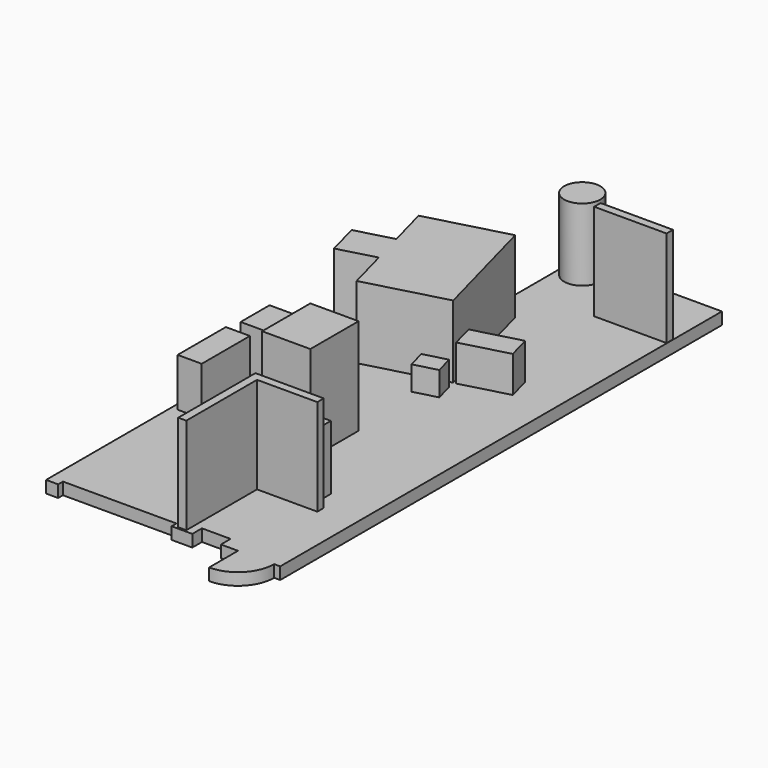
from build123d import *

# Parameters (mm, degrees)
F2_DEPTH  = 304.8
F3_DEPTH  = 1828.8
F4_DEPTH  = 914.4
F5_DEPTH  = 609.6
F6_DEPTH  = 2438.4
F1_W      = 1828.8
F1_H      = 203.2
F7_DEPTH  = 2438.4
F1_R      = 457.2
F8_DEPTH  = 1828.8
F1_W_2    = 1219.2
F1_H_2    = 1524
F10_DEPTH = 2438.4
F1_W_3    = 609.6
F11_DEPTH = 1219.2
F1_H_3    = 914.4
F12_DEPTH = 1270
F1_H_4    = 508
F13_DEPTH = 1625.6


# Not quite as in the source:
# - the program builds the solid bodies; features that only make, move or delete a surface that nothing else refers to are left out


with BuildPart() as f2:
    # F0 (on Top) → F2 (new body)
    with BuildSketch(Plane.XY):
        with BuildLine():
            Line((1349.4491028624, 7962.6567743872), (-631.7508971376, 7962.6567743872))
            Line((-631.7508971376, 7962.6567743872), (-631.7508971376, 5562.3567743872))
            Line((-631.7508971376, 5562.3567743872), (-2917.7508971376, 5562.3567743872))
            Line((-2917.7508971376, 5562.3567743872), (-2917.7508971376, 4292.3567743872))
            Line((-2917.7508971376, 4292.3567743872), (-2612.9508971376, 4292.3567743872))
            Line((-2612.9508971376, 4292.3567743872), (-2612.9508971376, 3898.6567743872))
            Line((-2612.9508971376, 3898.6567743872), (-2917.7508971376, 3898.6567743872))
            Line((-2917.7508971376, 3898.6567743872), (-2917.7508971376, -5994.6432256128))
            Line((-2917.7508971376, -5994.6432256128), (-2612.9508971376, -5994.6432256128))
            Line((-2612.9508971376, -5994.6432256128), (-2612.9508971376, -5842.2432256128))
            Line((-2612.9508971376, -5842.2432256128), (257.2491028624, -5842.2432256128))
            Line((257.2491028624, -5842.2432256128), (257.2491028624, -5994.6432256128))
            Line((257.2491028624, -5994.6432256128), (777.9491028624, -5994.6432256128))
            Line((777.9491028624, -5994.6432256128), (777.9491028624, -5689.8432256128))
            Line((777.9491028624, -5689.8432256128), (1501.8491028624, -5689.8432256128))
            Line((1501.8491028624, -5689.8432256128), (1501.8491028624, -5994.6432256128))
            Line((1501.8491028624, -5994.6432256128), (1933.6491028624, -5994.6432256128))
            Line((1933.6491028624, -5994.6432256128), (1933.6491028624, -6909.0432256128))
            ThreePointArc((1933.6491028624, -6909.0432256128), (2580.2275435794, -6641.2216663298), (2848.0491028624, -5994.6432256128))
            Line((2848.0491028624, -5994.6432256128), (3000.4491028624, -5994.6432256128))
            Line((3000.4491028624, -5994.6432256128), (3000.4491028624, 7962.6567743872))
            Line((3000.4491028624, 7962.6567743872), (1400.2491028624, 7962.6567743872))
            Line((1400.2491028624, 7962.6567743872), (1400.2491028624, 7872.949492893))
            Line((1400.2491028624, 7872.949492893), (1349.4491028624, 7872.949492893))
            Line((1349.4491028624, 7872.949492893), (1349.4491028624, 7962.6567743872))
        make_face()
    extrude(amount=-F2_DEPTH)

    # F1 (on face) → F3 (join)
    with BuildSketch(Plane.XY):
        Polygon((-26.2950770926, 5214.4638891469), (-2038.1253880874, 4675.3955820074), (-1755.4432270265, 3620.4113945345), (-2687.7548345607, 3370.5992522015), (-2464.2387072101, 2536.4257086183), (-1531.9270996759, 2786.2378509512), (-1249.2449386149, 1731.2536634783), (762.5853723799, 2270.3219706178), align=None)
    extrude(amount=F3_DEPTH)

    # F1 (on face) → F4 (join)
    with BuildSketch(Plane.XY):
        Polygon((1851.109756179, 3182.4776451945), (673.4529887674, 2866.9254654056), (831.2290786619, 2278.0970816997), (2008.8858460735, 2593.6492614887), align=None)
    extrude(amount=F4_DEPTH)

    # F1 (on face) → F5 (join)
    with BuildSketch(Plane.XY):
        Polygon((940.0834735112, 1607.8900389488), (815.1774023448, 2074.0458427159), (235.5625582244, 1918.7385133128), (360.4686293909, 1452.5827095457), align=None)
    extrude(amount=F5_DEPTH)

    # F1 (on face) → F6 (join)
    with BuildSketch(Plane.XY):
        Polygon((384.2491028624, -3507.7453807831), (384.2491028624, -5946.1453807831), (587.4491028624, -5946.1453807831), (587.4491028624, -3710.9453807831), (2111.4491028624, -3710.9453807831), (2111.4491028624, -3507.7453807831), (587.4491028624, -3507.7453807831), align=None)
    extrude(amount=F6_DEPTH)

    # F1 (on face) → F7 (join)
    with BuildSketch(Plane.XY):
        with Locations((2077.7624378014, 6325.4560646057)):
            Rectangle(F1_W, F1_H)
    extrude(amount=F7_DEPTH)

    # F1 (on face) → F8 (join)
    with BuildSketch(Plane.XY):
        with Locations((-123.7508971376, 7454.6567743872)):
            Circle(F1_R)
    extrude(amount=F8_DEPTH)

    # F1 (on face) → F10 (join)
    with BuildSketch(Plane.XY):
        with Locations((-22.1508971376, -1264.2254741287)):
            Rectangle(F1_W_2, F1_H_2)
    extrude(amount=F10_DEPTH)

    # F1 (on face) → F11 (join)
    with BuildSketch(Plane.XY):
        with Locations((-2460.5508971376, -1267.46)):
            Rectangle(F1_W_3, F1_H_2)
    extrude(amount=F11_DEPTH)

    # F1 (on face) → F12 (join)
    with BuildSketch(Plane.XY):
        with Locations((-1698.5508971376, 228.3567743872)):
            Rectangle(F1_W, F1_H_3)
    extrude(amount=F12_DEPTH)

    # F1 (on face) → F13 (join)
    with BuildSketch(Plane.XY):
        with Locations((1236.0154769325, -3205.4853807831)):
            Rectangle(F1_W_2, F1_H_4)
    extrude(amount=F13_DEPTH)


solid = f2.part
